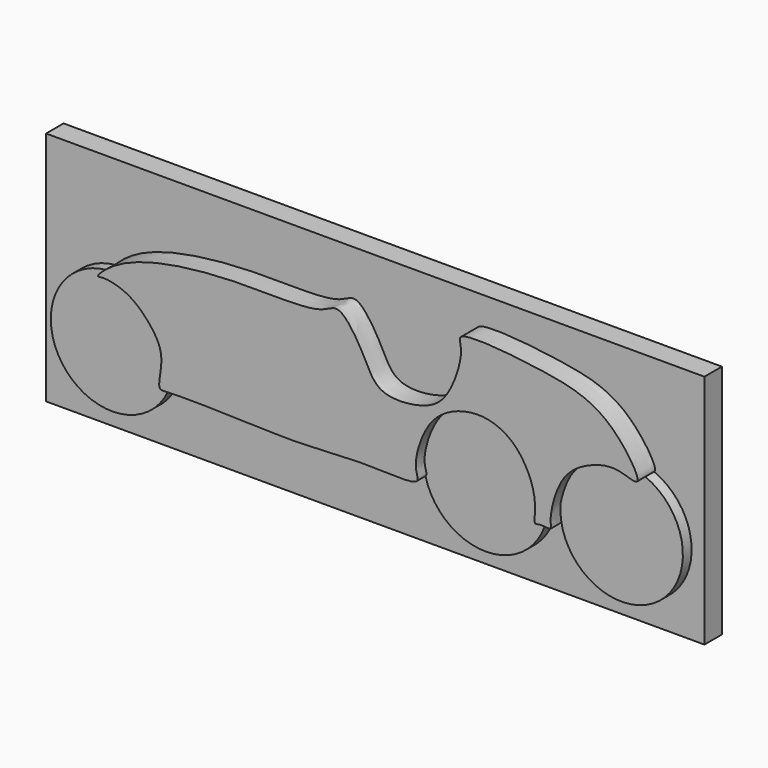
from build123d import *

# Parameters (mm, degrees)
F1_DEPTH = 5.08
F2_R     = 14.2693911651
F2_R_2   = 14.4913050141
F2_R_3   = 14.2149626285
F3_DEPTH = 2.54
F4_W     = 152.8010480106
F4_H     = 54.7436866909
F5_DEPTH = 5.08


with BuildPart() as f1:
    # F0 (on Front) → F1 (new body)
    with BuildSketch(Plane.XZ):
        with BuildLine():
            add(Edge.make_bspline(
                [(91.5712565184, -9.2397667468), (92.2506480563, -8.2749470462), (84.9113245453, 3.1798594145), (70.8467974857, 6.4181927802), (48.8332787058, 8.5309369462), (51.5486143438, 4.3017852457), (48.2016691437, -6.4469408419), (42.3635108736, -10.5530108465), (31.1184852851, -11.4295798728), (28.3687855118, -4.0550399622), (22.4675463664, 5.0385674737), (17.8382568777, 0.4935749268), (-2.2950387326, 2.115822892), (-27.0175658443, -1.0779135774), (-34.5321187873, -8.4627553793), (-32.1571834004, -7.7367093188), (-26.5137455595, -8.87129833), (-21.4443960259, -13.6708651421), (-17.8445998546, -19.3395019887), (-20.1391841532, -26.7293454582), (-16.8515502737, -26.297396327), (-1.1960392938, -26.4787884568), (14.5866665398, -27.230017872), (27.7107531727, -25.7764686423), (41.8998775602, -27.064060779), (39.5931139928, -23.2071559851), (41.3098684942, -16.1421466789), (45.400764541, -9.8084807721), (54.744677355, -6.4611988974), (64.1502761137, -10.1403721367), (68.6546470421, -20.2082352415), (67.3404925327, -26.0724056416), (68.9579468969, -25.1902033019), (72.0263382532, -25.8406484035), (70.9785957414, -23.8423375175), (73.2211458732, -13.5489426008), (80.4615197177, -9.1440319937), (86.8179947956, -7.6554584837), (91.1514306429, -9.8359712222), (91.5712565184, -9.2397667468)],
                knots=[0, 0, 0, 0, 0.032352452, 0.0733982234, 0.1147688033, 0.1296720721, 0.161259323, 0.1876682491, 0.2174747927, 0.2442187833, 0.2734302346, 0.2932689645, 0.3365877203, 0.3871354552, 0.4125249184, 0.4222866357, 0.4452987666, 0.4711419471, 0.4963737391, 0.5204253105, 0.5335074952, 0.5716439954, 0.6113678944, 0.6485816228, 0.6811183455, 0.695897892, 0.7217242331, 0.7483769579, 0.7776330933, 0.8072922446, 0.8393350268, 0.8598083045, 0.8698915329, 0.8853183596, 0.8960228644, 0.9265659292, 0.9547499904, 0.9800079987, 1, 1, 1, 1], degree=3))
        make_face()
    extrude(amount=F1_DEPTH)

    # F2 (on Front) → F3 (join)
    with BuildSketch(Plane.XZ):
        with Locations((-32.2942994535, -21.9899229705)):
            Circle(F2_R)
        with Locations((54.4311888516, -22.218964994)):
            Circle(F2_R_2)
        with Locations((85.9213247895, -22.4718973041)):
            Circle(F2_R_3)
    extrude(amount=F3_DEPTH)

    # F4 (on face) → F5 (join)
    with BuildSketch(Plane(origin=(0, 0, 0), x_dir=(-1, 0, 0), z_dir=(0, 1, 0))):
        with Locations((-26.7047379166, -13.5355284438)):
            Rectangle(F4_W, F4_H)
        with BuildLine():
            ThreePointArc((-71.7641032696, -21.1919592722), (-93.2496135528, -34.6522645534), (-91.4224704366, -9.3645497807))
            add(Edge.make_bspline(
                [(-91.4224704366, -9.3645497807), (-91.483438431, -9.3345677033), (-91.5334184104, -9.2935015226), (-91.5712565184, -9.2397667468)],
                knots=[0.9981981589, 0.9981981589, 0.9981981589, 0.9981981589, 1, 1, 1, 1], degree=3))
            add(Edge.make_bspline(
                [(-91.5712565184, -9.2397667468), (-92.2506480563, -8.2749470462), (-84.9113245453, 3.1798594145), (-70.8467974857, 6.4181927802), (-48.8332787058, 8.5309369462), (-51.5486143438, 4.3017852457), (-48.2016691437, -6.4469408419), (-42.3635108736, -10.5530108465), (-31.1184852851, -11.4295798728), (-28.3687855118, -4.0550399622), (-22.4675463664, 5.0385674737), (-17.8382568777, 0.4935749268), (2.2950387326, 2.115822892), (26.3423706651, -0.9906896679), (33.0882654966, -7.0685434619), (33.4823266027, -7.7700736143)],
                knots=[0, 0, 0, 0, 0.032352452, 0.0733982234, 0.1147688033, 0.1296720721, 0.161259323, 0.1876682491, 0.2174747927, 0.2442187833, 0.2734302346, 0.2932689645, 0.3365877203, 0.3871354552, 0.4092679276, 0.4092679276, 0.4092679276, 0.4092679276], degree=3))
            ThreePointArc((33.4823266027, -7.7700736143), (43.5049039677, -30.8181657542), (18.7493643013, -26.4788266165))
            add(Edge.make_bspline(
                [(18.7493643013, -26.4788266165), (18.4519204543, -26.5260702022), (15.7860916045, -26.3097412334), (1.1960392938, -26.4787884568), (-14.5866665398, -27.230017872), (-27.6841155442, -25.7794188746), (-39.3444353452, -26.8321842659), (-40.3982232078, -25.8347354863)],
                knots=[0.5266145409, 0.5266145409, 0.5266145409, 0.5266145409, 0.5335074952, 0.5716439954, 0.6113678944, 0.6485816228, 0.6808961481, 0.6808961481, 0.6808961481, 0.6808961481], degree=3))
            ThreePointArc((-40.3982232078, -25.8347354863), (-54.6019115257, -36.7092643277), (-68.545448318, -25.5031088285))
            add(Edge.make_bspline(
                [(-68.545448318, -25.5031088284), (-68.6704321284, -25.4783833949), (-69.5702113673, -25.3199926212), (-72.0263382532, -25.8406484035), (-71.3341318036, -24.5204350229), (-71.5239070275, -22.4163817486), (-71.7641032696, -21.1919592722)],
                knots=[0.8670345301, 0.8670345301, 0.8670345301, 0.8670345301, 0.8698915329, 0.8853183596, 0.8960228644, 0.9073343036, 0.9073343036, 0.9073343036, 0.9073343036], degree=3))
        make_face(mode=Mode.SUBTRACT)
        with BuildLine():
            add(Edge.make_bspline(
                [(-91.4224704366, -9.3645497807), (-91.483438431, -9.3345677033), (-91.5334184104, -9.2935015226), (-91.5712565184, -9.2397667468)],
                knots=[0.9981981589, 0.9981981589, 0.9981981589, 0.9981981589, 1, 1, 1, 1], degree=3))
            ThreePointArc((-91.4224704366, -9.3645497807), (-93.2496135528, -34.6522645534), (-71.7641032696, -21.1919592722))
            add(Edge.make_bspline(
                [(-68.545448318, -25.5031088284), (-68.6704321284, -25.4783833949), (-69.5702113673, -25.3199926212), (-72.0263382532, -25.8406484035), (-71.3341318036, -24.5204350229), (-71.5239070275, -22.4163817486), (-71.7641032696, -21.1919592722)],
                knots=[0.8670345301, 0.8670345301, 0.8670345301, 0.8670345301, 0.8698915329, 0.8853183596, 0.8960228644, 0.9073343036, 0.9073343036, 0.9073343036, 0.9073343036], degree=3))
            ThreePointArc((-68.545448318, -25.5031088285), (-54.6019115257, -36.7092643277), (-40.3982232078, -25.8347354863))
            add(Edge.make_bspline(
                [(18.7493643013, -26.4788266165), (18.4519204543, -26.5260702022), (15.7860916045, -26.3097412334), (1.1960392938, -26.4787884568), (-14.5866665398, -27.230017872), (-27.6841155442, -25.7794188746), (-39.3444353452, -26.8321842659), (-40.3982232078, -25.8347354863)],
                knots=[0.5266145409, 0.5266145409, 0.5266145409, 0.5266145409, 0.5335074952, 0.5716439954, 0.6113678944, 0.6485816228, 0.6808961481, 0.6808961481, 0.6808961481, 0.6808961481], degree=3))
            ThreePointArc((18.7493643013, -26.4788266165), (43.5049039677, -30.8181657542), (33.4823266027, -7.7700736143))
            add(Edge.make_bspline(
                [(-91.5712565184, -9.2397667468), (-92.2506480563, -8.2749470462), (-84.9113245453, 3.1798594145), (-70.8467974857, 6.4181927802), (-48.8332787058, 8.5309369462), (-51.5486143438, 4.3017852457), (-48.2016691437, -6.4469408419), (-42.3635108736, -10.5530108465), (-31.1184852851, -11.4295798728), (-28.3687855118, -4.0550399622), (-22.4675463664, 5.0385674737), (-17.8382568777, 0.4935749268), (2.2950387326, 2.115822892), (26.3423706651, -0.9906896679), (33.0882654966, -7.0685434619), (33.4823266027, -7.7700736143)],
                knots=[0, 0, 0, 0, 0.032352452, 0.0733982234, 0.1147688033, 0.1296720721, 0.161259323, 0.1876682491, 0.2174747927, 0.2442187833, 0.2734302346, 0.2932689645, 0.3365877203, 0.3871354552, 0.4092679276, 0.4092679276, 0.4092679276, 0.4092679276], degree=3))
        make_face()
        with BuildLine():
            add(Edge.make_bspline(
                [(-49.6714292893, -8.531649336), (-51.2410951526, -7.9559168443), (-54.5268632955, -7.3196207082), (-57.7214051638, -7.9363725541), (-59.1681431159, -8.5237400849)],
                knots=[0.7618743813, 0.7618743813, 0.7618743813, 0.7618743813, 0.7776330933, 0.7923343894, 0.7923343894, 0.7923343894, 0.7923343894], degree=3))
            ThreePointArc((-49.6714292893, -8.531649336), (-54.4191199052, -7.7276650056), (-59.1681431159, -8.5237400849))
        make_face(mode=Mode.SUBTRACT)
    extrude(amount=F5_DEPTH)


solid = f1.part
